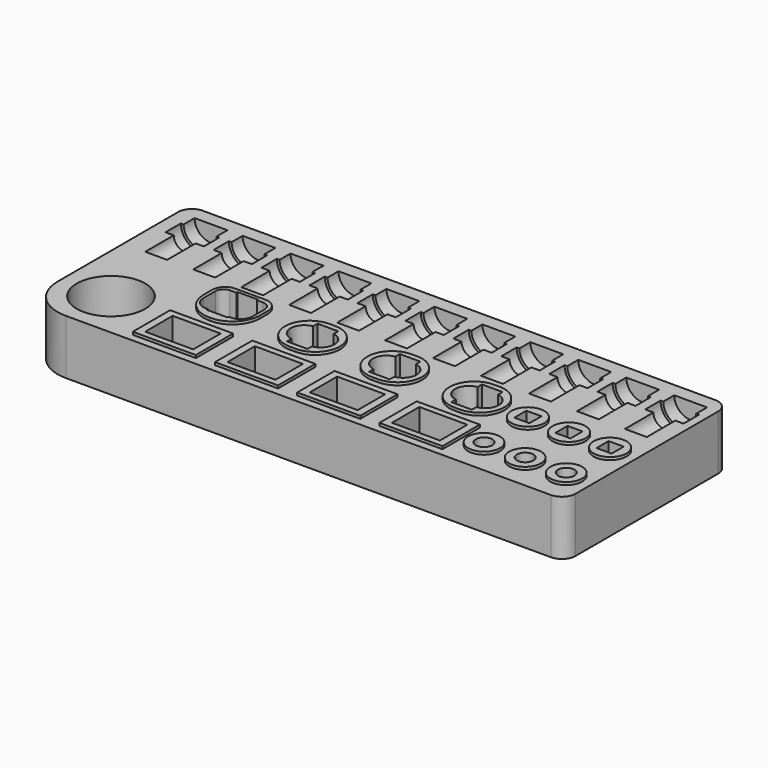
from build123d import *

# Parameters (mm, degrees)
F0_R          = 12.5
F1_DEPTH      = 20
F14_W         = 17.5
F14_H         = 12.5
F15_DEPTH     = 8
F14_W_2       = 23
F14_H_2       = 17
F16_DEPTH     = 1
F18_DEPTH     = 19
F19_DEPTH     = 1
F20_R         = 6
F20_W         = 5.5
F20_H         = 5.5
F20_R_2       = 5.8
F20_R_3       = 3
F21_DEPTH     = 1
F22_DEPTH     = 8
F23_DEPTH     = 10.5
F24_TEXT_SIZE = 5.5555555556
F25_DEPTH     = 1


# Not quite as in the source:
# - Text() gives the source's letters only with a copy of the font that has no kerning and outlines rounded to 1/6400 em; it was checked with that copy


with BuildPart() as f1:
    # F0 (on Top) → F1 (new body)
    with BuildSketch(Plane.XY):
        with BuildLine():
            ThreePointArc((0, 15), (4.3933982822, 4.3933982822), (15, 0))
            Line((15, 0), (192, 0))
            ThreePointArc((192, 0), (195.5355339059, 1.4644660941), (197, 5))
            Line((197, 5), (197, 70))
            ThreePointArc((197, 70), (195.5355339059, 73.5355339059), (192, 75))
            Line((192, 75), (5, 75))
            ThreePointArc((5, 75), (1.4644660941, 73.5355339059), (0, 70))
            Line((0, 70), (0, 15))
        make_face()
        with Locations((17.5, 17.5)):
            Circle(F0_R, mode=Mode.SUBTRACT)
    extrude(amount=F1_DEPTH)

    # F2 (on face) → F3 (revolve, cut)
    with BuildSketch(Plane.XY.offset(20)):
        Polygon((18, 70), (12, 70), (12, 65), (12, 58), (12, 45), (16, 45), (16, 58), (19, 58), (19, 65), (18, 65), align=None)
    revolve(axis=Axis((12, 51.5, 20), (0, -1, 0)), mode=Mode.SUBTRACT)

    # F2 (on face) → F4 (revolve, cut)
    with BuildSketch(Plane.XY.offset(20)):
        Polygon((35.5, 70), (29.5, 70), (29.5, 65), (29.5, 58), (29.5, 45), (33.5, 45), (33.5, 58), (36.5, 58), (36.5, 65), (35.5, 65), align=None)
    revolve(axis=Axis((29.5, 51.5, 20), (0, -1, 0)), mode=Mode.SUBTRACT)

    # F2 (on face) → F5 (revolve, cut)
    with BuildSketch(Plane.XY.offset(20)):
        Polygon((53, 70), (47, 70), (47, 65), (47, 58), (47, 45), (51, 45), (51, 58), (54, 58), (54, 65), (53, 65), align=None)
    revolve(axis=Axis((47, 51.5, 20), (0, -1, 0)), mode=Mode.SUBTRACT)

    # F2 (on face) → F6 (revolve, cut)
    with BuildSketch(Plane.XY.offset(20)):
        Polygon((70.5, 70), (64.5, 70), (64.5, 65), (64.5, 58), (64.5, 45), (68.5, 45), (68.5, 58), (71.5, 58), (71.5, 65), (70.5, 65), align=None)
    revolve(axis=Axis((64.5, 51.5, 20), (0, -1, 0)), mode=Mode.SUBTRACT)

    # F2 (on face) → F7 (revolve, cut)
    with BuildSketch(Plane.XY.offset(20)):
        Polygon((88, 70), (82, 70), (82, 65), (82, 58), (82, 45), (86, 45), (86, 58), (89, 58), (89, 65), (88, 65), align=None)
    revolve(axis=Axis((82, 51.5, 20), (0, -1, 0)), mode=Mode.SUBTRACT)

    # F2 (on face) → F8 (revolve, cut)
    with BuildSketch(Plane.XY.offset(20)):
        Polygon((105.5, 70), (99.5, 70), (99.5, 65), (99.5, 58), (99.5, 45), (103.5, 45), (103.5, 58), (106.5, 58), (106.5, 65), (105.5, 65), align=None)
    revolve(axis=Axis((99.5, 51.5, 20), (0, -1, 0)), mode=Mode.SUBTRACT)

    # F2 (on face) → F9 (revolve, cut)
    with BuildSketch(Plane.XY.offset(20)):
        Polygon((123, 70), (117, 70), (117, 65), (117, 58), (117, 45), (121, 45), (121, 58), (124, 58), (124, 65), (123, 65), align=None)
    revolve(axis=Axis((117, 51.5, 20), (0, -1, 0)), mode=Mode.SUBTRACT)

    # F2 (on face) → F10 (revolve, cut)
    with BuildSketch(Plane.XY.offset(20)):
        Polygon((140.5, 70), (134.5, 70), (134.5, 65), (134.5, 58), (134.5, 45), (138.5, 45), (138.5, 58), (141.5, 58), (141.5, 65), (140.5, 65), align=None)
    revolve(axis=Axis((134.5, 51.5, 20), (0, -1, 0)), mode=Mode.SUBTRACT)

    # F2 (on face) → F11 (revolve, cut)
    with BuildSketch(Plane.XY.offset(20)):
        Polygon((175.5, 70), (169.5, 70), (169.5, 65), (169.5, 58), (169.5, 45), (173.5, 45), (173.5, 58), (176.5, 58), (176.5, 65), (175.5, 65), align=None)
    revolve(axis=Axis((169.5, 51.5, 20), (0, -1, 0)), mode=Mode.SUBTRACT)

    # F2 (on face) → F12 (revolve, cut)
    with BuildSketch(Plane.XY.offset(20)):
        Polygon((158, 70), (152, 70), (152, 65), (152, 58), (152, 45), (156, 45), (156, 58), (159, 58), (159, 65), (158, 65), align=None)
    revolve(axis=Axis((152, 51.5, 20), (0, -1, 0)), mode=Mode.SUBTRACT)

    # F2 (on face) → F13 (revolve, cut)
    with BuildSketch(Plane.XY.offset(20)):
        Polygon((193, 70), (187, 70), (187, 65), (187, 58), (187, 45), (191, 45), (191, 58), (194, 58), (194, 65), (193, 65), align=None)
    revolve(axis=Axis((187, 51.5, 20), (0, -1, 0)), mode=Mode.SUBTRACT)

    # F14 (on face) → F15 (cut)
    with BuildSketch(Plane.XY.offset(20)):
        with Locations((48.75, 11.25)):
            Rectangle(F14_W, F14_H)
        with Locations((78.75, 11.25)):
            Rectangle(F14_W, F14_H)
        with Locations((108.75, 11.25)):
            Rectangle(F14_W, F14_H)
        with Locations((138.75, 11.25)):
            Rectangle(F14_W, F14_H)
    extrude(amount=-F15_DEPTH, mode=Mode.SUBTRACT)

    # F14 (on face) → F16 (join)
    with BuildSketch(Plane.XY.offset(20)):
        with Locations((78.75, 11.25)):
            Rectangle(F14_W_2, F14_H_2)
        with Locations((78.75, 11.25)):
            Rectangle(F14_W, F14_H, mode=Mode.SUBTRACT)
        with Locations((108.75, 11.25)):
            Rectangle(F14_W_2, F14_H_2)
        with Locations((108.75, 11.25)):
            Rectangle(F14_W, F14_H, mode=Mode.SUBTRACT)
        with Locations((138.75, 11.25)):
            Rectangle(F14_W_2, F14_H_2)
        with Locations((138.75, 11.25)):
            Rectangle(F14_W, F14_H, mode=Mode.SUBTRACT)
        with Locations((48.75, 11.25)):
            Rectangle(F14_W_2, F14_H_2)
        with Locations((48.75, 11.25)):
            Rectangle(F14_W, F14_H, mode=Mode.SUBTRACT)
    extrude(amount=F16_DEPTH)

    # F17 (on face) → F18 (cut)
    with BuildSketch(Plane.XY.offset(20)):
        with BuildLine():
            ThreePointArc((40, 31.5), (41.3180194847, 28.3180194847), (44.5, 27))
            Line((44.5, 27), (45.25, 27))
            Line((45.25, 27), (45.25, 26.5))
            Line((45.25, 26.5), (52.75, 26.5))
            Line((52.75, 26.5), (52.75, 27))
            Line((52.75, 27), (53.5, 27))
            ThreePointArc((53.5, 27), (56.6819805153, 28.3180194847), (58, 31.5))
            Line((58, 31.5), (58, 37))
            ThreePointArc((58, 37), (57.1213203436, 39.1213203436), (55, 40))
            Line((55, 40), (52.75, 40))
            Line((52.75, 40), (52.75, 40.5))
            Line((52.75, 40.5), (45.25, 40.5))
            Line((45.25, 40.5), (45.25, 40))
            Line((45.25, 40), (43, 40))
            ThreePointArc((43, 40), (40.8786796564, 39.1213203436), (40, 37))
            Line((40, 37), (40, 31.5))
        make_face()
        with BuildLine():
            Line((82.7502346946, 37.4676514922), (82.7502346946, 39.5242215088))
            Line((82.7502346946, 39.5242215088), (75.2502346946, 39.5242215088))
            Line((75.2502346946, 39.5242215088), (75.2502346946, 37.4676514922))
            ThreePointArc((75.2502346946, 37.4676514922), (71.0002346946, 32.5242215088), (75.2502346946, 27.5807915255))
            Line((75.2502346946, 27.5807915255), (75.2502346946, 25.5242215088))
            Line((75.2502346946, 25.5242215088), (82.7502346946, 25.5242215088))
            Line((82.7502346946, 25.5242215088), (82.7502346946, 27.5242215088))
            Line((82.7502346946, 27.5242215088), (82.7502346946, 27.5807915255))
            ThreePointArc((82.7502346946, 27.5807915255), (87.0002346946, 32.5242215088), (82.7502346946, 37.4676514922))
        make_face()
        with BuildLine():
            Line((112.7502346946, 37.4676514922), (112.7502346946, 39.5242215088))
            Line((112.7502346946, 39.5242215088), (105.2502346946, 39.5242215088))
            Line((105.2502346946, 39.5242215088), (105.2502346946, 37.4676514922))
            ThreePointArc((105.2502346946, 37.4676514922), (101.0002346946, 32.5242215088), (105.2502346946, 27.5807915255))
            Line((105.2502346946, 27.5807915255), (105.2502346946, 25.5242215088))
            Line((105.2502346946, 25.5242215088), (112.7502346946, 25.5242215088))
            Line((112.7502346946, 25.5242215088), (112.7502346946, 27.5807915255))
            ThreePointArc((112.7502346946, 27.5807915255), (117.0002346946, 32.5242215088), (112.7502346946, 37.4676514922))
        make_face()
        with BuildLine():
            Line((142.7502346946, 37.4676514922), (142.7502346946, 39.5242215088))
            Line((142.7502346946, 39.5242215088), (135.2502346946, 39.5242215088))
            Line((135.2502346946, 39.5242215088), (135.2502346946, 37.4676514922))
            ThreePointArc((135.2502346946, 37.4676514922), (131.0002346946, 32.5242215088), (135.2502346946, 27.5807915255))
            Line((135.2502346946, 27.5807915255), (135.2502346946, 27.5242215088))
            Line((135.2502346946, 27.5242215088), (135.2502346946, 25.5242215088))
            Line((135.2502346946, 25.5242215088), (142.7502346946, 25.5242215088))
            Line((142.7502346946, 25.5242215088), (142.7502346946, 27.5807915255))
            ThreePointArc((142.7502346946, 27.5807915255), (147.0002346946, 32.5242215088), (142.7502346946, 37.4676514922))
        make_face()
    extrude(amount=-F18_DEPTH, mode=Mode.SUBTRACT)

    # F17 (on face) → F19 (join)
    with BuildSketch(Plane.XY.offset(20)):
        with BuildLine():
            Line((48.7502346946, 23.2742215088), (49.2502346946, 23.2742215088))
            ThreePointArc((49.2502346946, 23.2742215088), (56.3213025065, 26.203153697), (59.2502346946, 33.2742215088))
            Line((59.2502346946, 33.2742215088), (59.2502346946, 37.0242215088))
            ThreePointArc((59.2502346946, 37.0242215088), (57.8589919053, 40.3829787195), (54.5002346946, 41.7742215088))
            Line((54.5002346946, 41.7742215088), (43.5002346946, 41.7742215088))
            ThreePointArc((43.5002346946, 41.7742215088), (40.141477484, 40.3829787195), (38.7502346946, 37.0242215088))
            Line((38.7502346946, 37.0242215088), (38.7502346946, 33.2742215088))
            ThreePointArc((38.7502346946, 33.2742215088), (41.6791668828, 26.203153697), (48.7502346946, 23.2742215088))
        make_face()
        with BuildLine():
            Line((45.25, 27), (44.5, 27))
            ThreePointArc((44.5, 27), (41.3180194847, 28.3180194847), (40, 31.5))
            Line((40, 31.5), (40, 37))
            ThreePointArc((40, 37), (40.8786796564, 39.1213203436), (43, 40))
            Line((43, 40), (45.25, 40))
            Line((45.25, 40), (45.25, 40.5))
            Line((45.25, 40.5), (52.75, 40.5))
            Line((52.75, 40.5), (52.75, 40))
            Line((52.75, 40), (55, 40))
            ThreePointArc((55, 40), (57.1213203436, 39.1213203436), (58, 37))
            Line((58, 37), (58, 31.5))
            ThreePointArc((58, 31.5), (56.6819805153, 28.3180194847), (53.5, 27))
            Line((53.5, 27), (52.75, 27))
            Line((52.75, 27), (52.75, 26.5))
            Line((52.75, 26.5), (45.25, 26.5))
            Line((45.25, 26.5), (45.25, 27))
        make_face(mode=Mode.SUBTRACT)
        with BuildLine():
            ThreePointArc((78.0002346946, 41.5242215088), (69.0002346946, 32.5242215088), (78.0002346946, 23.5242215088))
            Line((78.0002346946, 23.5242215088), (80.0002346946, 23.5242215088))
            ThreePointArc((80.0002346946, 23.5242215088), (89.0002346946, 32.5242215088), (80.0002346946, 41.5242215088))
            Line((80.0002346946, 41.5242215088), (78.0002346946, 41.5242215088))
        make_face()
        with BuildLine():
            Line((75.2502346946, 39.5242215088), (82.7502346946, 39.5242215088))
            Line((82.7502346946, 39.5242215088), (82.7502346946, 37.4676514922))
            ThreePointArc((82.7502346946, 37.4676514922), (87.0002346946, 32.5242215088), (82.7502346946, 27.5807915255))
            Line((82.7502346946, 27.5807915255), (82.7502346946, 27.5242215088))
            Line((82.7502346946, 27.5242215088), (82.7502346946, 25.5242215088))
            Line((82.7502346946, 25.5242215088), (75.2502346946, 25.5242215088))
            Line((75.2502346946, 25.5242215088), (75.2502346946, 27.5807915255))
            ThreePointArc((75.2502346946, 27.5807915255), (71.0002346946, 32.5242215088), (75.2502346946, 37.4676514922))
            Line((75.2502346946, 37.4676514922), (75.2502346946, 39.5242215088))
        make_face(mode=Mode.SUBTRACT)
        with BuildLine():
            Line((110.0002346946, 41.5242215088), (108.0002346946, 41.5242215088))
            ThreePointArc((108.0002346946, 41.5242215088), (99.0002346946, 32.5242215088), (108.0002346946, 23.5242215088))
            Line((108.0002346946, 23.5242215088), (110.0002346946, 23.5242215088))
            ThreePointArc((110.0002346946, 23.5242215088), (119.0002346946, 32.5242215088), (110.0002346946, 41.5242215088))
        make_face()
        with BuildLine():
            Line((105.2502346946, 39.5242215088), (112.7502346946, 39.5242215088))
            Line((112.7502346946, 39.5242215088), (112.7502346946, 37.4676514922))
            ThreePointArc((112.7502346946, 37.4676514922), (117.0002346946, 32.5242215088), (112.7502346946, 27.5807915255))
            Line((112.7502346946, 27.5807915255), (112.7502346946, 25.5242215088))
            Line((112.7502346946, 25.5242215088), (105.2502346946, 25.5242215088))
            Line((105.2502346946, 25.5242215088), (105.2502346946, 27.5807915255))
            ThreePointArc((105.2502346946, 27.5807915255), (101.0002346946, 32.5242215088), (105.2502346946, 37.4676514922))
            Line((105.2502346946, 37.4676514922), (105.2502346946, 39.5242215088))
        make_face(mode=Mode.SUBTRACT)
        with BuildLine():
            Line((140.0002346946, 41.5242215088), (138.0002346946, 41.5242215088))
            ThreePointArc((138.0002346946, 41.5242215088), (129.0002346946, 32.5242215088), (138.0002346946, 23.5242215088))
            Line((138.0002346946, 23.5242215088), (140.0002346946, 23.5242215088))
            ThreePointArc((140.0002346946, 23.5242215088), (149.0002346946, 32.5242215088), (140.0002346946, 41.5242215088))
        make_face()
        with BuildLine():
            Line((135.2502346946, 39.5242215088), (142.7502346946, 39.5242215088))
            Line((142.7502346946, 39.5242215088), (142.7502346946, 37.4676514922))
            ThreePointArc((142.7502346946, 37.4676514922), (147.0002346946, 32.5242215088), (142.7502346946, 27.5807915255))
            Line((142.7502346946, 27.5807915255), (142.7502346946, 25.5242215088))
            Line((142.7502346946, 25.5242215088), (135.2502346946, 25.5242215088))
            Line((135.2502346946, 25.5242215088), (135.2502346946, 27.5242215088))
            Line((135.2502346946, 27.5242215088), (135.2502346946, 27.5807915255))
            ThreePointArc((135.2502346946, 27.5807915255), (131.0002346946, 32.5242215088), (135.2502346946, 37.4676514922))
            Line((135.2502346946, 37.4676514922), (135.2502346946, 39.5242215088))
        make_face(mode=Mode.SUBTRACT)
    extrude(amount=F19_DEPTH)

    # F20 (on face) → F21 (join)
    with BuildSketch(Plane.XY.offset(20)):
        with Locations((158, 32)):
            Circle(F20_R)
        with Locations((158, 32)):
            Rectangle(F20_W, F20_H, mode=Mode.SUBTRACT)
        with Locations((173, 32)):
            Circle(F20_R)
        with Locations((173, 32)):
            Rectangle(F20_W, F20_H, mode=Mode.SUBTRACT)
        with Locations((188, 32)):
            Circle(F20_R)
        with Locations((188, 32)):
            Rectangle(F20_W, F20_H, mode=Mode.SUBTRACT)
        with Locations((188, 12)):
            Circle(F20_R_2)
        with Locations((188, 12)):
            Circle(F20_R_3, mode=Mode.SUBTRACT)
        with Locations((173, 12)):
            Circle(F20_R_2)
        with Locations((173, 12)):
            Circle(F20_R_3, mode=Mode.SUBTRACT)
        with Locations((158, 12)):
            Circle(F20_R_2)
        with Locations((158, 12)):
            Circle(F20_R_3, mode=Mode.SUBTRACT)
    extrude(amount=F21_DEPTH)

    # F20 (on face) → F22 (cut)
    with BuildSketch(Plane.XY.offset(20)):
        with Locations((158, 32)):
            Rectangle(F20_W, F20_H)
        with Locations((173, 32)):
            Rectangle(F20_W, F20_H)
        with Locations((188, 32)):
            Rectangle(F20_W, F20_H)
    extrude(amount=-F22_DEPTH, mode=Mode.SUBTRACT)

    # F20 (on face) → F23 (cut)
    with BuildSketch(Plane.XY.offset(20)):
        with Locations((158, 12)):
            Circle(F20_R_3)
        with Locations((173, 12)):
            Circle(F20_R_3)
        with Locations((188, 12)):
            Circle(F20_R_3)
    extrude(amount=-F23_DEPTH, mode=Mode.SUBTRACT)

    # F24 (on face) → F25 (cut)
    with BuildSketch(Plane(origin=(0, 0, 0), x_dir=(1, 0, 0), z_dir=(0, 0, -1))):
        with Locations((30, -9)):
            Text('876, 882', F24_TEXT_SIZE, font='Open Sans', text_align=(TextAlign.LEFT, TextAlign.BOTTOM))
    extrude(amount=F25_DEPTH, mode=Mode.SUBTRACT)


solid = f1.part
